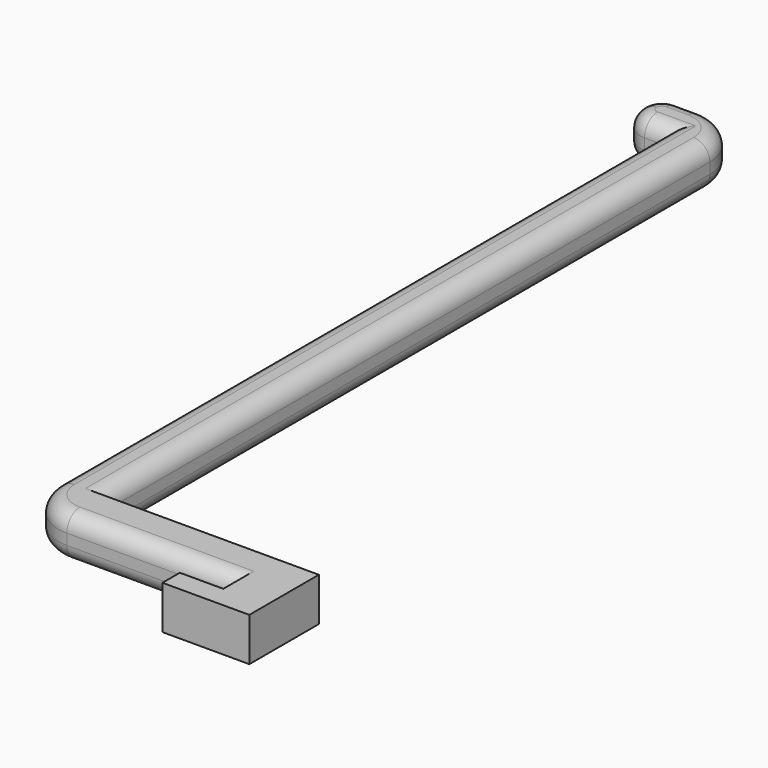
from build123d import *

# Parameters (mm, degrees)
F1_DEPTH = 4
F2_R     = 1.5


# Not quite as in the source:
# - ends of sketch curves that miss each other by under 0.0002 mm in the source are joined


with BuildPart() as f1:
    # F0 (on Top) → F1 (new body)
    with BuildSketch(Plane.XY):
        with BuildLine():
            Line((-5.7822973108, 10.3064593036), (-5.7822973108, 0))
            Line((-5.7822973108, 0), (-5.7822973108, -59.6935572128))
            ThreePointArc((-5.7822973108, -59.6935572128), (-4.6107244356, -62.5219843376), (-1.7822973108, -63.6935572128))
            Line((-1.7822973108, -63.6935572128), (14.2177026892, -63.6935572128))
            Line((14.2177026892, -63.6935572128), (14.2177026892, -65.6935572128))
            Line((14.2177026892, -65.6935572128), (10.2177026892, -65.6935572128))
            Line((10.2177026892, -65.6935572128), (10.2177026892, -67.6935572128))
            Line((10.2177026892, -67.6935572128), (18.2177026892, -67.6935572128))
            Line((18.2177026892, -67.6935572128), (18.2177026892, -59.6935572128))
            Line((18.2177026892, -59.6935572128), (-1.7822973108, -59.6935572128))
            Line((-1.7822973108, -59.6935572128), (-1.7822973108, 10.3064427872))
            ThreePointArc((-1.7822973108, 10.3064427872), (-2.9538701861, 13.1348699119), (-5.7822973108, 14.3064427872))
            Line((-5.7822973108, 14.3064427872), (-7.7880364463, 14.3064427872))
            ThreePointArc((-7.7880364463, 14.3064427872), (-9.2042805699, 13.7186228687), (-9.7880281881, 12.3006953697))
            ThreePointArc((-9.7880281881, 12.3006953697), (-9.2002165753, 10.8902151801), (-7.7880364938, 10.3064593036))
            Line((-7.7880364938, 10.3064593036), (-5.7822973108, 10.3064593036))
        make_face()
    extrude(amount=F1_DEPTH)

    # F2
    f2_edges = [f1.edges().sort_by_distance(p)[0] for p in [
        (-5.782297, -24.693549, 4),
        (-1.782297, -24.693557, 4),
        (-2.95387, 13.13487, 4),
        (-6.785167, 14.306443, 4),
        (-9.204281, 13.718623, 4),
        (-9.200211, 10.890209, 4),
        (-6.785167, 10.306459, 4),
        (-1.782297, -24.693557, 0),
        (-2.95387, 13.13487, 0),
        (-6.785167, 14.306443, 0),
        (-9.204281, 13.718623, 0),
        (-9.200211, 10.890209, 0),
        (-6.785167, 10.306459, 0),
        (-5.782297, -24.693549, 0),
    ]]
    fillet(f2_edges, radius=F2_R)


solid = f1.part
